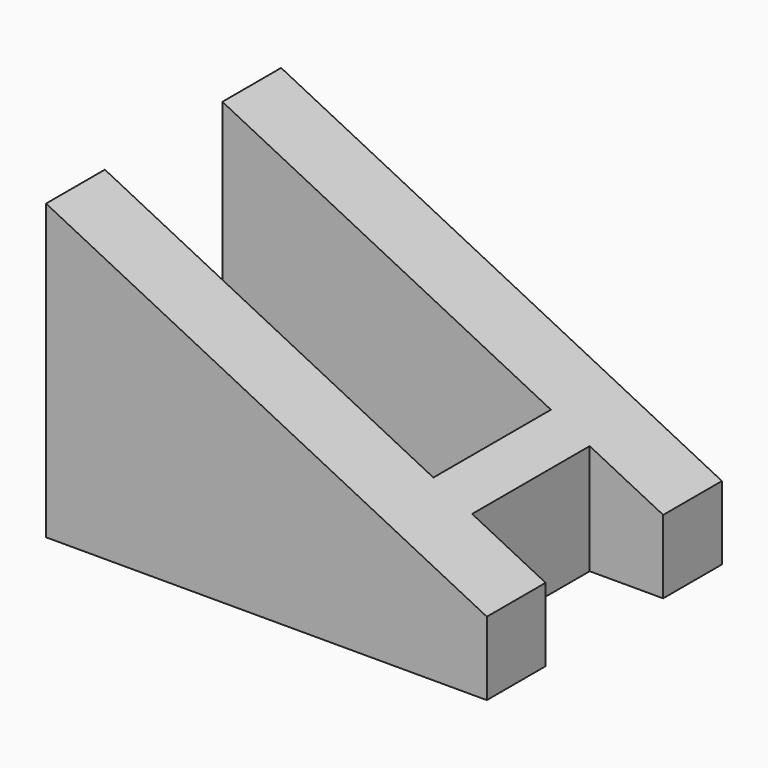
from build123d import *

# Parameters (mm, degrees)
F1_DEPTH = 20
F2_W     = 25
F2_H     = 10
F3_DEPTH = 10
F4_W     = 10
F4_H     = 5
F4_H_2   = 2.5
F5_DEPTH = 5


with BuildPart() as f1:
    # F0 (on Front) → F1 (new body)
    with BuildSketch(Plane.XZ):
        Polygon((30, 5), (0, 20), (0, 0), (30, 0), align=None)
    extrude(amount=-F1_DEPTH)

    # F2 (on face) → F3 (cut)
    with BuildSketch(Plane(origin=(8, 0, 16), x_dir=(0.894427191, 0, -0.4472135955), z_dir=(0.4472135955, 0, 0.894427191))):
        with Locations((3.55572809, 10)):
            Rectangle(F2_W, F2_H)
    extrude(amount=-F3_DEPTH, mode=Mode.SUBTRACT)

    # F4 (on face) → F5 (cut)
    with BuildSketch(Plane.YZ.offset(30)):
        with Locations((10, 2.5)):
            Rectangle(F4_W, F4_H)
        with Locations((10, 6.25)):
            Rectangle(F4_W, F4_H_2)
    extrude(amount=-F5_DEPTH, mode=Mode.SUBTRACT)


solid = f1.part
